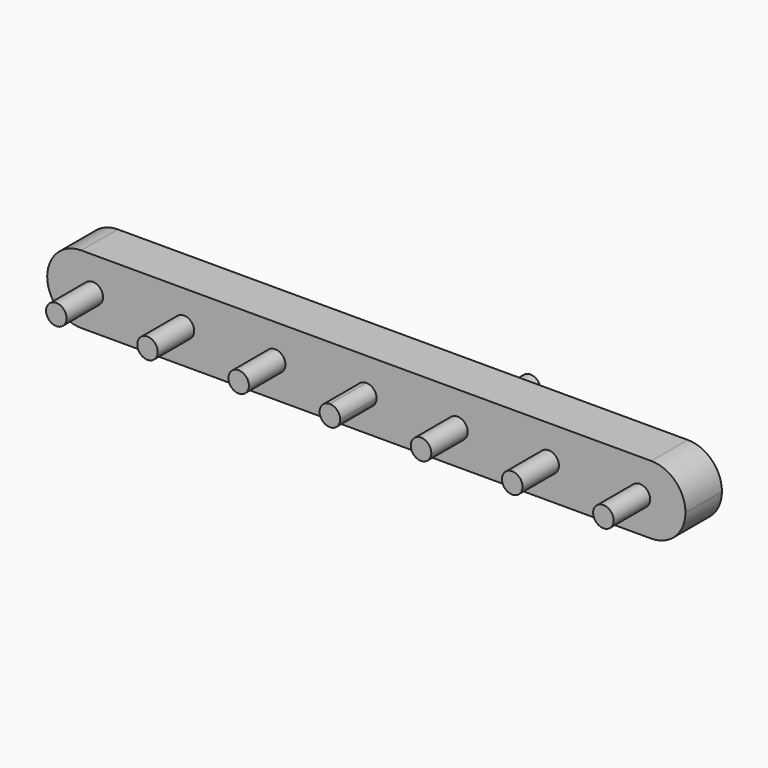
from build123d import *

# Parameters (mm, degrees)
F0_R     = 2.8575
F1_DEPTH = 12.7
F2_DEPTH = 25.4
F3_R     = 2.8575
F4_DEPTH = 12.7
F5_R     = 9.52499


# Not quite as in the source:
# - a fillet or chamfer is up to 0.001 mm smaller than in the source, because OpenCascade refuses the exact size
# - a feature names something its author has since deleted; it is built from what else it names


with BuildPart() as f1:
    # F0 (on Front) → F1 (new body)
    with BuildSketch(Plane.XZ):
        Polygon((-88.9, -9.525), (88.9, -9.525), (88.9, 9.525), (0, 9.525), (-88.9, 9.525), align=None)
        with Locations((-76.2, 0)):
            Circle(F0_R, mode=Mode.SUBTRACT)
        with Locations((-50.8, 0)):
            Circle(F0_R, mode=Mode.SUBTRACT)
        with Locations((-25.4, 0)):
            Circle(F0_R, mode=Mode.SUBTRACT)
        with BuildLine():
            ThreePointArc((2.8575, 0), (-2.0205576272, -2.0205576272), (0, 2.8575))
            ThreePointArc((0, 2.8575), (2.0205576272, 2.0205576272), (2.8575, 0))
        make_face(mode=Mode.SUBTRACT)
        with Locations((25.4, 0)):
            Circle(F0_R, mode=Mode.SUBTRACT)
        with Locations((50.8, 0)):
            Circle(F0_R, mode=Mode.SUBTRACT)
        with Locations((76.2, 0)):
            Circle(F0_R, mode=Mode.SUBTRACT)
    extrude(amount=F1_DEPTH)

    # F0 (on Front) → F2 (join)
    with BuildSketch(Plane.XZ):
        with BuildLine():
            ThreePointArc((2.8575, 0), (2.0205576272, 2.0205576272), (0, 2.8575))
            ThreePointArc((0, 2.8575), (-2.0205576272, -2.0205576272), (2.8575, 0))
        make_face()
        with Locations((-76.2, 0)):
            Circle(F0_R)
        with Locations((-50.8, 0)):
            Circle(F0_R)
        with Locations((-25.4, 0)):
            Circle(F0_R)
        with Locations((25.4, 0)):
            Circle(F0_R)
        with Locations((50.8, 0)):
            Circle(F0_R)
        with Locations((76.2, 0)):
            Circle(F0_R)
    extrude(amount=F2_DEPTH)

    # F3 (on face) → F4 (join)
    with BuildSketch(Plane(origin=(0, 0, 0), x_dir=(-1, 0, 0), z_dir=(0, 1, 0))):
        with Locations((-25.4, 0)):
            Circle(F3_R)
    extrude(amount=F4_DEPTH)

    # F5 (radius 9.525 in the source; OpenCascade refuses exactly that, so slightly less here)
    f5_edges = [f1.edges().sort_by_distance(p)[0] for p in [
        (88.9, -6.35, 9.525),
        (88.9, -6.35, -9.525),
        (-88.9, -6.35, -9.525),
        (-88.9, -6.35, 9.525),
    ]]
    fillet(f5_edges, radius=F5_R)


solid = f1.part
